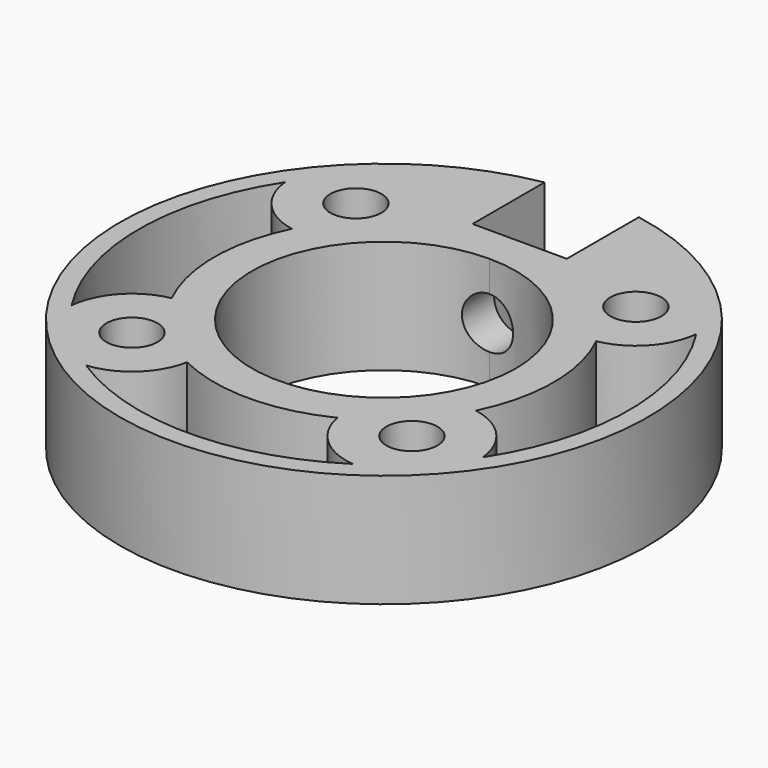
from build123d import *

# Parameters (mm, degrees)
F0_R            = 2.15265
F1_DEPTH        = 9.525
F2_R            = 2.15265
F3_REACH        = 42.6021136501
F5_R            = 3.96875
F6_DEPTH        = 3.175
F8_DEPTH        = 9.525
F8_COPIES_COUNT = 3
F8_COPIES_ANGLE = 180


# Not quite as in the source:
# - a pattern or mirror of a feature is missing from the dataset's text; its kind, count and spacing are read off the source's solid


with BuildPart() as f1:
    # F0 (on Top) → F1 (new body)
    with BuildSketch(Plane.XY):
        with BuildLine():
            Line((3.96875, 14.2875), (0, 14.2875))
            Line((0, 14.2875), (-3.96875, 14.2875))
            Line((-3.96875, 14.2875), (-3.96875, 21.8677764859))
            ThreePointArc((-3.96875, 21.8677764859), (0, -22.225), (3.96875, 21.8677764859))
            Line((3.96875, 21.8677764859), (3.96875, 14.2875))
        make_face()
        with Locations((-11.7865861589, -11.7865861589)):
            Circle(F0_R, mode=Mode.SUBTRACT)
        with Locations((11.7865861589, -11.7865861589)):
            Circle(F0_R, mode=Mode.SUBTRACT)
        with Locations((-11.7865861589, 11.7865861589)):
            Circle(F0_R, mode=Mode.SUBTRACT)
        with BuildLine():
            ThreePointArc((0, 11.1125), (7.8577241059, 7.8577241059), (11.1125, 0))
            ThreePointArc((11.1125, 0), (-7.8577241059, -7.8577241059), (0, 11.1125))
        make_face(mode=Mode.SUBTRACT)
        with Locations((11.7865861589, 11.7865861589)):
            Circle(F0_R, mode=Mode.SUBTRACT)
    extrude(amount=F1_DEPTH)

    f3_end = f1.faces().sort_by_distance((0, -11.1125, 4.7625))[0]
    # F2 (on face) → F3 (cut, up to a face of the model that its end follows)
    with BuildSketch(Plane(origin=(0, 14.2875, 0), x_dir=(-1, 0, 0), z_dir=(0, 1, 0))):
        with Locations((0, 4.7625)):
            Circle(F2_R)
    f3_long = extrude(amount=-F3_REACH, mode=Mode.PRIVATE)
    add(split(f3_long, bisect_by=f3_end, keep=Keep.ALL, mode=Mode.PRIVATE).solids().sort_by_distance((0, 14.2875, 4.7625))[0], mode=Mode.SUBTRACT)

    # F5 (on face) → F6 (cut, through all)
    with BuildSketch(Plane(origin=(0, 0, 0), x_dir=(1, 0, 0), z_dir=(0, 0, -1))):
        with Locations((11.7865861589, -11.7865861589)):
            Circle(F5_R)
        with Locations((-11.7865861589, 11.7865861589)):
            Circle(F5_R)
    extrude(amount=-F6_DEPTH, mode=Mode.SUBTRACT)

    # F7 (on face) → F8 (cut, through all)
    with BuildSketch(Plane(origin=(0, 0, 0), x_dir=(1, 0, 0), z_dir=(0, 0, -1))):
        with BuildLine():
            ThreePointArc((-17.3148424047, -11.229543123), (-15.8788163052, -8.0281867), (-12.8109235396, -6.3255746232))
            ThreePointArc((-12.8109235396, -6.3255746232), (-14.2875, 0), (-12.8109235396, 6.3255746232))
            ThreePointArc((-12.8109235396, 6.3255746232), (-15.8788163052, 8.0281867), (-17.3148424047, 11.229543123))
            ThreePointArc((-17.3148424047, 11.229543123), (-20.6375, 0), (-17.3148424047, -11.229543123))
        make_face()
    f8 = extrude(amount=-F8_DEPTH, mode=Mode.SUBTRACT)

    # F8_copies: F8 ×3 about axis
    f8_copies_axis = Axis((0, 0, 0), (0, 0, 1))
    for i in range(1, F8_COPIES_COUNT):
        add(f8.rotate(f8_copies_axis, i * F8_COPIES_ANGLE / (F8_COPIES_COUNT - 1)), mode=Mode.SUBTRACT)


solid = f1.part
